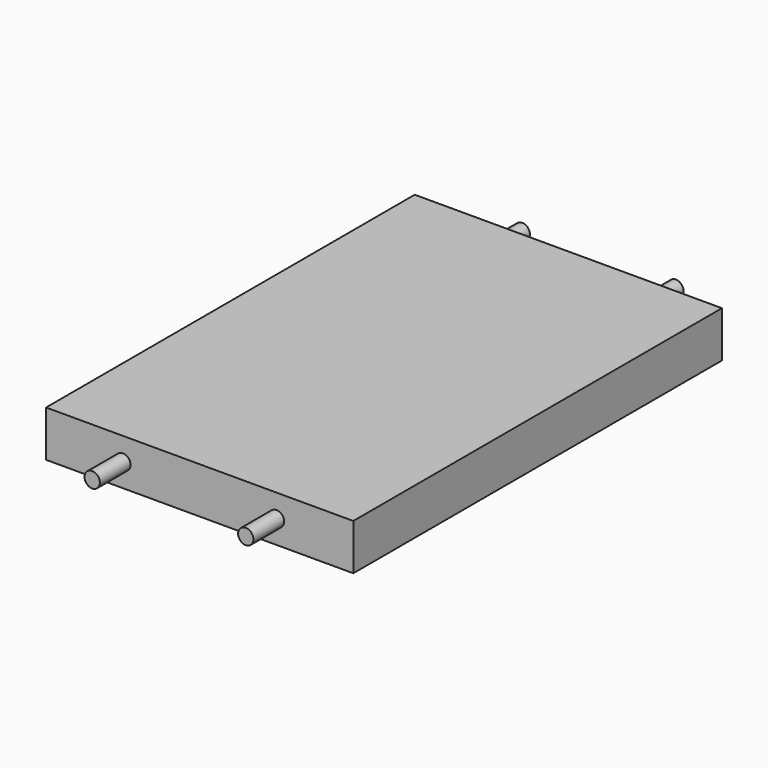
from build123d import *

# Parameters (mm, degrees)
F2_DEPTH = 45
F3_R     = 44.9999
F0_R     = 50
F4_DEPTH = 1500
F5_DEPTH = 1750


# Not quite as in the source:
# - a fillet or chamfer is up to 0.001 mm smaller than in the source, because OpenCascade refuses the exact size
# - a feature names something its author has since deleted; it is built from what else it names


with BuildPart() as f1:
    # F0 (on Front) → F1 (revolve)
    with BuildSketch(Plane.XZ):
        Polygon((53.877471291, 45), (-16.122528709, 22.5), (53.877471291, 22.5), align=None)
        Polygon((-16.122528709, 22.5), (0, 0), (53.877471291, 0), (53.877471291, 22.5), align=None)
        Polygon((-86.1157540445, 0), (0, 0), (-16.122528709, 22.5), (-102.2382827536, 22.5), align=None)
    revolve(axis=Axis((-43.0578770223, 0, 0), (1, 0, 0)))

    # F0 (on Front) → F2 (join, symmetric)
    with BuildSketch(Plane.XZ):
        Polygon((53.877471291, 22.5), (53.877471291, 0), (53.877471291, -45), (146.2954133749, -45), (198.256937602, 45), (198.256937602, 251.7713010311), (78.877471291, 45), (53.877471291, 45), align=None)
    extrude(amount=F2_DEPTH, both=True)

    # F3 (radius 45 in the source; OpenCascade refuses exactly that, so slightly less here)
    f3_edges = [f1.edges().sort_by_distance(p)[0] for p in [
        (100.086442, 45, -45),
        (100.086442, -45, -45),
    ]]
    fillet(f3_edges, radius=F3_R)


with BuildPart() as f4:
    # F0 (on Front) → F4 (new body, symmetric)
    with BuildSketch(Plane.XZ):
        Polygon((198.256937602, 345), (198.256937602, 251.7713010311), (198.256937602, 45), (2198.256937602, 45), (2198.256937602, 135), (2198.256937602, 345), align=None)
        with Locations((698.256937602, 195)):
            Circle(F0_R, mode=Mode.SUBTRACT)
        with Locations((1698.256937602, 195)):
            Circle(F0_R, mode=Mode.SUBTRACT)
    extrude(amount=F4_DEPTH, both=True)

    # F0 (on Front) → F5 (join, symmetric)
    with BuildSketch(Plane.XZ):
        with Locations((1698.256937602, 195)):
            Circle(F0_R)
        with Locations((698.256937602, 195)):
            Circle(F0_R)
    extrude(amount=F5_DEPTH, both=True)


solid = Compound([f1.part, f4.part])
